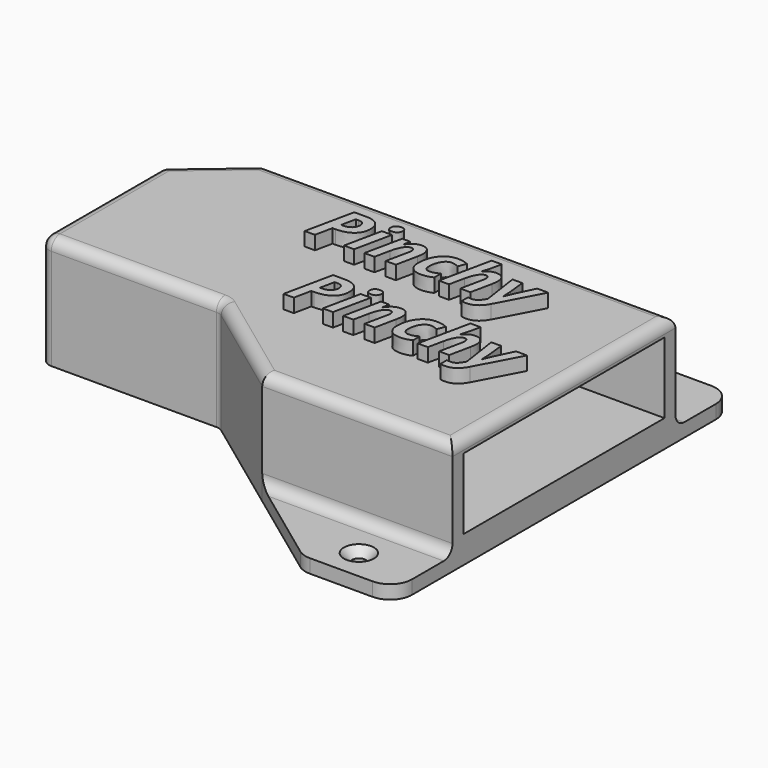
from build123d import *

# Parameters (mm, degrees)
F1_DEPTH        = 22.86
F2_T            = -3.175
F4_DEPTH        = 3.175
F5_R            = 2.54
F6_TEXT_SIZE    = 15.941631036
F7_DEPTH        = 3.175
F9_R            = 5.08
F10_D           = 3.175
F10_CSINK_D     = 6.985
F10_CSINK_ANGLE = 90


# Not quite as in the source:
# - Text() gives the source's letters only with a copy of the font that has no kerning and outlines rounded to 1/6400 em; it was checked with that copy


with BuildPart() as f1:
    # F0 (on Top) → F1 (new body)
    with BuildSketch(Plane.XY):
        Polygon((-79.0451991608, -3.175), (-37.2887030571, -3.175), (-13.4309201095, -20.735535543), (30.7868943831, -20.735535543), (30.7868943831, 44.034464457), (-64.9930103204, 44.034464457), (-79.0451991608, 32.1297015951), align=None)
    extrude(amount=F1_DEPTH)

    # F2
    f2_openings = [f1.faces().sort_by_distance(p)[0] for p in [
        (30.786894, 11.649464, 11.43),
    ]]
    offset(amount=F2_T, openings=f2_openings, kind=Kind.INTERSECTION)

    # F3 (on face) → F4 (join)
    with BuildSketch(Plane(origin=(0, 0, 0), x_dir=(1, 0, 0), z_dir=(0, 0, -1))):
        Polygon((-79.0451991608, 3.175), (-79.0451991608, -32.1297015951), (-45.1301024695, -60.861964457), (30.7868943831, -60.861964457), (30.7868943831, 37.575735543), (9.448213355, 37.575735543), (-13.4309201095, 20.735535543), (-37.2887030571, 3.175), align=None)
    extrude(amount=F4_DEPTH)

    # F5
    f5_edges = [f1.edges().sort_by_distance(p)[0] for p in [
        (-17.103058, 44.034464, 0),
        (-17.103058, 44.034464, 22.86),
        (-58.166951, -3.175, 22.86),
        (-25.359812, -11.955268, 22.86),
        (8.677987, -20.735536, 22.86),
        (30.786894, 11.649464, 22.86),
        (-72.019105, 38.082083, 22.86),
        (-79.045199, 14.477351, 22.86),
        (8.677987, -20.735536, 0),
        (-79.045199, -3.175, 9.8425),
        (-79.045199, 32.129702, 9.8425),
        (-37.288703, -3.175, 9.8425),
    ]]
    fillet(f5_edges, radius=F5_R)

    # F6 (on face) → F7 (join)
    with BuildSketch(Plane.XY.offset(22.86)):
        with Locations((-39.1169059465, 23.200441549)):
            Text('Pinchy', F6_TEXT_SIZE, font='Open Sans', font_style=FontStyle.BOLDITALIC, text_align=(TextAlign.LEFT, TextAlign.BOTTOM))
        with Locations((-26.689906378, 1.5198233401)):
            Text('Pinchy', F6_TEXT_SIZE, font='Open Sans', font_style=FontStyle.BOLDITALIC, text_align=(TextAlign.LEFT, TextAlign.BOTTOM))
    extrude(amount=F7_DEPTH)

    # F9
    f9_edges = [f1.edges().sort_by_distance(p)[0] for p in [
        (-45.130102, 60.861964, -1.5875),
        (30.786894, 60.861964, -1.5875),
        (30.786894, -37.575736, -1.5875),
        (9.448213, -37.575736, -1.5875),
    ]]
    fillet(f9_edges, radius=F9_R)

    # F10 (through all)
    with Locations(Plane.XY):
        with Locations((-38.4718887508, 53.724564457), (16.8010108173, 53.724564457), (16.8010108173, -30.438335543)):
            CounterSinkHole(F10_D / 2, F10_CSINK_D / 2, counter_sink_angle=F10_CSINK_ANGLE)


solid = f1.part
